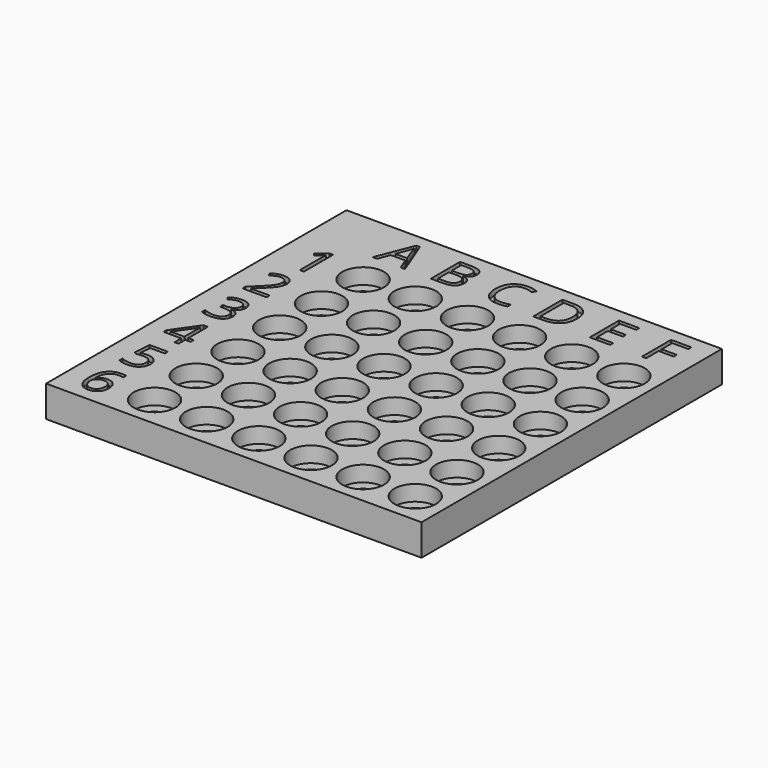
from build123d import *

# Parameters (mm, degrees)
F0_W           = 114.3
F0_H           = 114.3
F1_DEPTH       = 9.525
F3_D           = 6.35
F3_DEPTH       = 6.35
F3_CBORE_D     = 12.7
F3_CBORE_DEPTH = 4.7625
F3_TIP         = 1.9077324654
F4_TEXT_SIZE   = 15.5222222222
F5_DEPTH       = 1.5875


# Not quite as in the source:
# - Text() gives the source's letters only with a copy of the font that has no kerning and outlines rounded to 1/6400 em; it was checked with that copy


with BuildPart() as f1:
    # F0 (on Top) → F1 (new body)
    with BuildSketch(Plane.XY):
        with Locations((57.15, 57.15)):
            Rectangle(F0_W, F0_H)
    extrude(amount=F1_DEPTH)

    # F3
    with Locations(Plane.XY.offset(9.525)):
        with Locations((25.4, 88.9), (41.275, 88.9), (57.15, 88.9), (73.025, 88.9), (88.9, 88.9), (104.775, 88.9), (104.775, 73.025), (88.9, 73.025), (73.025, 73.025), (57.15, 73.025), (41.275, 73.025), (25.4, 73.025), (25.4, 57.15), (41.275, 57.15), (57.15, 57.15), (73.025, 57.15), (88.9, 57.15), (104.775, 57.15), (104.775, 41.275), (88.9, 41.275), (73.025, 41.275), (57.15, 41.275), (41.275, 41.275), (25.4, 41.275), (25.4, 25.4), (41.275, 25.4), (57.15, 25.4), (73.025, 25.4), (88.9, 25.4), (104.775, 25.4), (88.9, 9.525), (73.025, 9.525), (57.15, 9.525), (104.775, 9.525), (41.275, 9.525), (25.4, 9.525)):
            CounterBoreHole(F3_D / 2, F3_CBORE_D / 2, F3_CBORE_DEPTH, depth=F3_DEPTH)
            with Locations((0, 0, -(F3_DEPTH + F3_TIP / 2))):  # 118° drill point
                Cone(0, F3_D / 2, F3_TIP, mode=Mode.SUBTRACT)

    # F4 (on face) → F5 (cut)
    with BuildSketch(Plane.XY.offset(9.525)):
        with Locations((6.4297057292, 83.312)):
            Text('1', F4_TEXT_SIZE, font='Open Sans', text_align=(TextAlign.LEFT, TextAlign.BOTTOM))
        with Locations((5.1175928819, 67.437)):
            Text('2', F4_TEXT_SIZE, font='Open Sans', text_align=(TextAlign.LEFT, TextAlign.BOTTOM))
        with Locations((5.1563984375, 51.562)):
            Text('3', F4_TEXT_SIZE, font='Open Sans', text_align=(TextAlign.LEFT, TextAlign.BOTTOM))
        with Locations((4.8568680556, 35.687)):
            Text('4', F4_TEXT_SIZE, font='Open Sans', text_align=(TextAlign.LEFT, TextAlign.BOTTOM))
        with Locations((5.1479097222, 19.812)):
            Text('5', F4_TEXT_SIZE, font='Open Sans', text_align=(TextAlign.LEFT, TextAlign.BOTTOM))
        with Locations((5.08, 3.937)):
            Text('6', F4_TEXT_SIZE, font='Open Sans', text_align=(TextAlign.LEFT, TextAlign.BOTTOM))
        with Locations((19.9854123264, 99.314)):
            Text('A', F4_TEXT_SIZE, font='Open Sans', text_align=(TextAlign.LEFT, TextAlign.BOTTOM))
        with Locations((36.1708567708, 99.314)):
            Text('B', F4_TEXT_SIZE, font='Open Sans', text_align=(TextAlign.LEFT, TextAlign.BOTTOM))
        with Locations((51.9815850694, 99.314)):
            Text('C', F4_TEXT_SIZE, font='Open Sans', text_align=(TextAlign.LEFT, TextAlign.BOTTOM))
        with Locations((67.3375607639, 99.314)):
            Text('D', F4_TEXT_SIZE, font='Open Sans', text_align=(TextAlign.LEFT, TextAlign.BOTTOM))
        with Locations((84.5465017361, 99.314)):
            Text('E', F4_TEXT_SIZE, font='Open Sans', text_align=(TextAlign.LEFT, TextAlign.BOTTOM))
        with Locations((100.4215017361, 99.314)):
            Text('F', F4_TEXT_SIZE, font='Open Sans', text_align=(TextAlign.LEFT, TextAlign.BOTTOM))
    extrude(amount=-F5_DEPTH, mode=Mode.SUBTRACT)


solid = f1.part
